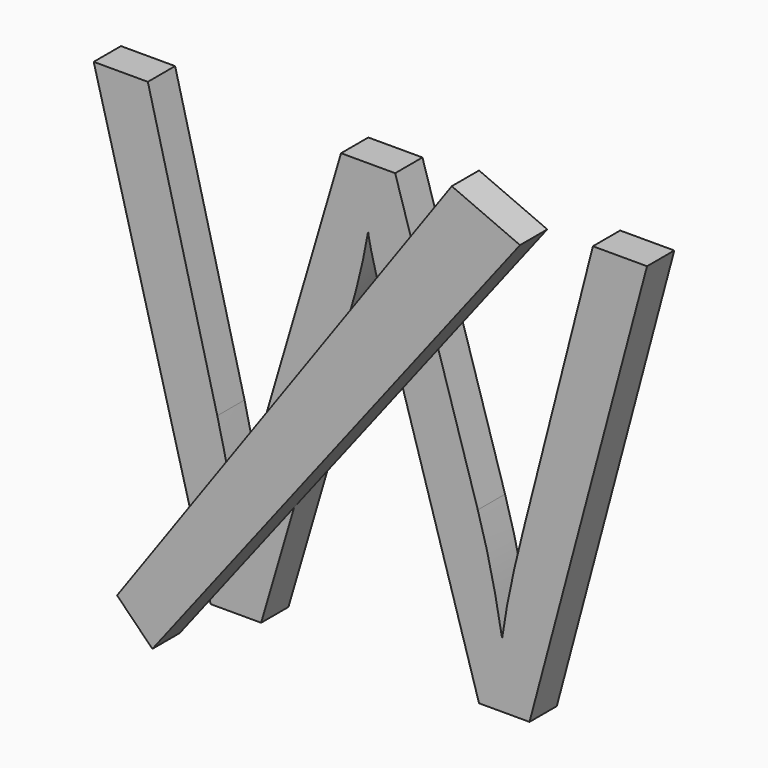
from build123d import *

# Parameters (mm, degrees)
F0_TEXT_SIZE = 90.2756298375
F1_DEPTH     = 5
F3_DEPTH     = 5


# Not quite as in the source:
# - Text() gives the source's letters only with a copy of the font that has no kerning and outlines rounded to 1/6400 em; it was checked with that copy


with BuildPart() as f1:
    # F0 (on Front) → F1 (new body)
    with BuildSketch(Plane.XZ):
        with Locations((-24.7602239251, -35.7491485775)):
            Text('W', F0_TEXT_SIZE, font='Open Sans', text_align=(TextAlign.LEFT, TextAlign.BOTTOM))
    extrude(amount=F1_DEPTH)

    # F2 (on face) → F3 (join)
    with BuildSketch(Plane.XZ.offset(5)):
        Polygon((32.9456513351, 33.0536775291), (-16.1460358649, -35.7491485775), (-10.9671186656, -40.9743711352), (42.9545491934, 28.6991877862), align=None)
    extrude(amount=F3_DEPTH)


solid = f1.part
